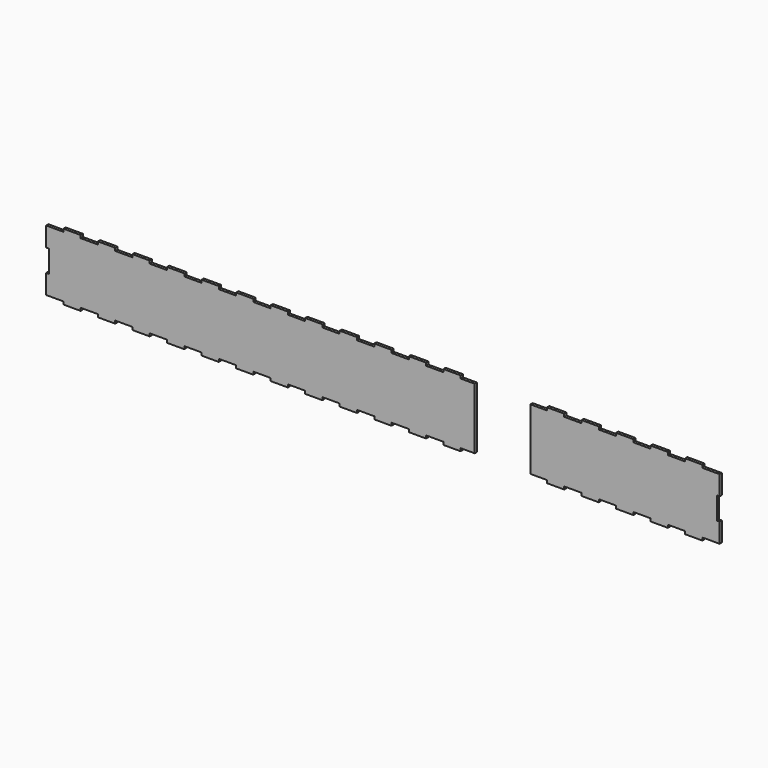
from build123d import *

# Parameters (mm, degrees)
F1_DEPTH = 3.175


# Not quite as in the source:
# - ends of sketch curves that miss each other by under 0.0002 mm in the source are joined


with BuildPart() as f1:
    # F0 (on Front) → F1 (new body)
    with BuildSketch(Plane.XZ):
        Polygon((-384.175, 34.925), (-384.175, 12.7), (-381, 12.7), (-381, -12.7), (-384.175, -12.7), (-384.175, -34.925), (-364.473717838, -34.925), (-364.473717838, -38.1), (-344.772435676, -38.1), (-344.772435676, -34.925), (-325.071153514, -34.925), (-325.071153514, -38.1), (-305.369871352, -38.1), (-305.369871352, -34.925), (-285.66858919, -34.925), (-285.66858919, -38.1), (-265.967307028, -38.1), (-265.967307028, -34.925), (-246.266024866, -34.925), (-246.266024866, -38.1), (-226.564742704, -38.1), (-226.564742704, -34.925), (-206.863460542, -34.925), (-206.863460542, -38.1), (-187.16217838, -38.1), (-187.16217838, -34.925), (-167.460896218, -34.925), (-167.460896218, -38.1), (-147.759614056, -38.1), (-147.759614056, -34.925), (-128.058331894, -34.925), (-128.058331894, -38.1), (-108.357049732, -38.1), (-108.357049732, -34.925), (-88.65576757, -34.925), (-88.65576757, -38.1), (-68.954485408, -38.1), (-68.954485408, -34.925), (-49.253203246, -34.925), (-49.253203246, -38.1), (-29.551921084, -38.1), (-29.551921084, -34.925), (-9.850638922, -34.925), (-9.850638922, -38.1), (9.85064324, -38.1), (9.85064324, -34.925), (29.551925402, -34.925), (29.551925402, -38.1), (49.253207564, -38.1), (49.253207564, -34.925), (68.954489726, -34.925), (68.954489726, -38.1), (88.655771888, -38.1), (88.655771888, -34.925), (104.775, -34.925), (104.775, 34.925), (88.655771888, 34.925), (88.655771888, 38.1), (68.954489726, 38.1), (68.954489726, 34.925), (49.253207564, 34.925), (49.253207564, 38.1), (29.551925402, 38.1), (29.551925402, 34.925), (9.85064324, 34.925), (9.85064324, 38.1), (-9.850638922, 38.1), (-9.850638922, 34.925), (-29.551921084, 34.925), (-29.551921084, 38.1), (-49.253203246, 38.1), (-49.253203246, 34.925), (-68.954485408, 34.925), (-68.954485408, 38.1), (-88.65576757, 38.1), (-88.65576757, 34.925), (-108.357049732, 34.925), (-108.357049732, 38.1), (-128.058331894, 38.1), (-128.058331894, 34.925), (-147.759614056, 34.925), (-147.759614056, 38.1), (-167.460896218, 38.1), (-167.460896218, 34.925), (-187.16217838, 34.925), (-187.16217838, 38.1), (-206.863460542, 38.1), (-206.863460542, 34.925), (-226.564742704, 34.925), (-226.564742704, 38.1), (-246.266024866, 38.1), (-246.266024866, 34.925), (-265.967307028, 34.925), (-265.967307028, 38.1), (-285.66858919, 38.1), (-285.66858919, 34.925), (-305.369871352, 34.925), (-305.369871352, 38.1), (-325.071153514, 38.1), (-325.071153514, 34.925), (-344.772435676, 34.925), (-344.772435676, 38.1), (-364.473717838, 38.1), (-364.473717838, 34.925), align=None)
    extrude(amount=F1_DEPTH)


with BuildPart() as f1b:
    # F0 (on Front) → F1, piece 2 (new body)
    with BuildSketch(Plane.XZ):
        Polygon((187.162182698, 34.925), (168.275, 34.925), (168.275, -34.925), (187.162182698, -34.925), (187.162182698, -38.1), (206.86346486, -38.1), (206.86346486, -34.925), (226.564747022, -34.925), (226.564747022, -38.1), (246.266029184, -38.1), (246.266029184, -34.925), (265.967311346, -34.925), (265.967311346, -38.1), (285.668593508, -38.1), (285.668593508, -34.925), (305.36987567, -34.925), (305.36987567, -38.1), (325.071157832, -38.1), (325.071157832, -34.925), (344.772439994, -34.925), (344.772439994, -38.1), (364.473722156, -38.1), (364.473722156, -34.925), (384.175004318, -34.925), (384.175, -12.7), (381, -12.7), (381, 12.7), (384.175, 12.7), (384.175, 34.925), (364.473722156, 34.925), (364.473722156, 38.1), (344.772439994, 38.1), (344.772439994, 34.925), (325.071157832, 34.925), (325.071157832, 38.1), (305.36987567, 38.1), (305.36987567, 34.925), (285.668593508, 34.925), (285.668593508, 38.1), (265.967311346, 38.1), (265.967311346, 34.925), (246.266029184, 34.925), (246.266029184, 38.1), (226.564747022, 38.1), (226.564747022, 34.925), (206.86346486, 34.925), (206.86346486, 38.1), (187.162182698, 38.1), align=None)
    extrude(amount=F1_DEPTH)


solid = Compound([f1.part, f1b.part])
